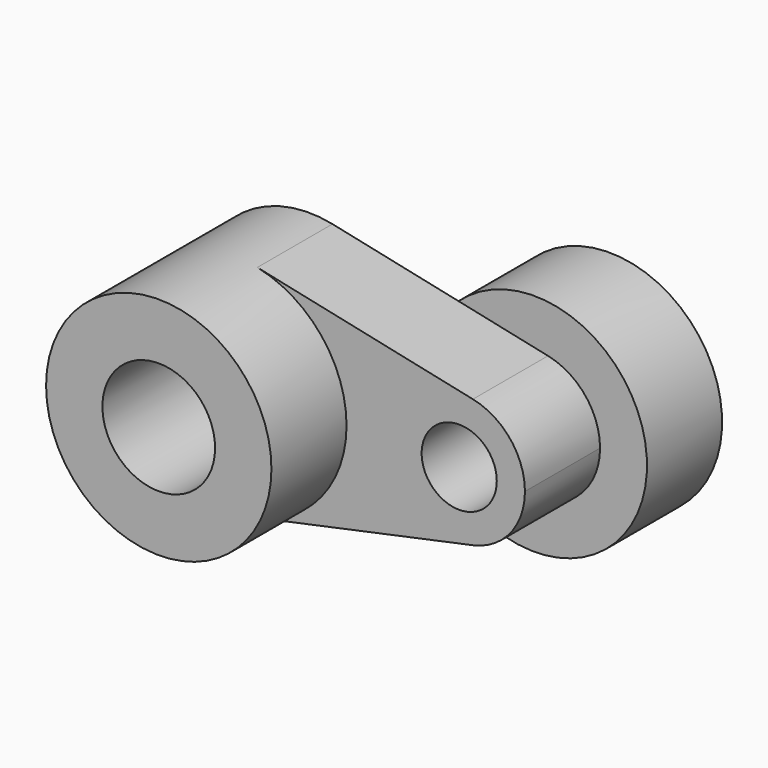
from build123d import *

# Parameters (mm, degrees)
F0_R     = 15
F0_R_2   = 10
F1_DEPTH = 25
F2_DEPTH = 50
F3_R     = 30
F3_R_2   = 10
F4_DEPTH = 25


# Not quite as in the source:
# - a feature names something its author has since deleted; it is built from what else it names


with BuildPart() as f1:
    # F0 (on Front) → F1 (new body)
    with BuildSketch(Plane.XZ):
        with BuildLine():
            ThreePointArc((6.25, -29.3417364858), (23.3184476327, -18.8745860882), (30, 0))
            ThreePointArc((30, 0), (23.3184476327, 18.8745860882), (6.25, 29.3417364858))
            ThreePointArc((6.25, 29.3417364858), (-30, 0), (6.25, -29.3417364858))
        make_face()
        Circle(F0_R, mode=Mode.SUBTRACT)
        with BuildLine():
            ThreePointArc((6.25, 29.3417364858), (23.3184476327, 18.8745860882), (30, 0))
            ThreePointArc((30, 0), (23.3184476327, -18.8745860882), (6.25, -29.3417364858))
            Line((6.25, -29.3417364858), (63.6458333333, -17.11601295))
            ThreePointArc((63.6458333333, -17.11601295), (42.5, 0), (63.6458333333, 17.11601295))
            Line((63.6458333333, 17.11601295), (6.25, 29.3417364858))
        make_face()
        with BuildLine():
            ThreePointArc((77.5, 0), (73.6024277858, 11.0101752181), (63.6458333333, 17.11601295))
            ThreePointArc((63.6458333333, 17.11601295), (42.5, 0), (63.6458333333, -17.11601295))
            ThreePointArc((63.6458333333, -17.11601295), (73.6024277858, -11.0101752181), (77.5, 0))
        make_face()
        with Locations((60, 0)):
            Circle(F0_R_2, mode=Mode.SUBTRACT)
    extrude(amount=F1_DEPTH)

    # F0 (on Front) → F2 (join)
    with BuildSketch(Plane.XZ):
        with BuildLine():
            ThreePointArc((6.25, -29.3417364858), (23.3184476327, -18.8745860882), (30, 0))
            ThreePointArc((30, 0), (23.3184476327, 18.8745860882), (6.25, 29.3417364858))
            ThreePointArc((6.25, 29.3417364858), (-30, 0), (6.25, -29.3417364858))
        make_face()
        Circle(F0_R, mode=Mode.SUBTRACT)
    extrude(amount=F2_DEPTH)

    # F3 (on face) → F4 (join)
    with BuildSketch(Plane(origin=(0, 0, 0), x_dir=(-1, 0, 0), z_dir=(0, 1, 0))):
        with Locations((-60, 0)):
            Circle(F3_R)
        with Locations((-60, 0)):
            Circle(F3_R_2, mode=Mode.SUBTRACT)
    extrude(amount=F4_DEPTH)


solid = f1.part
